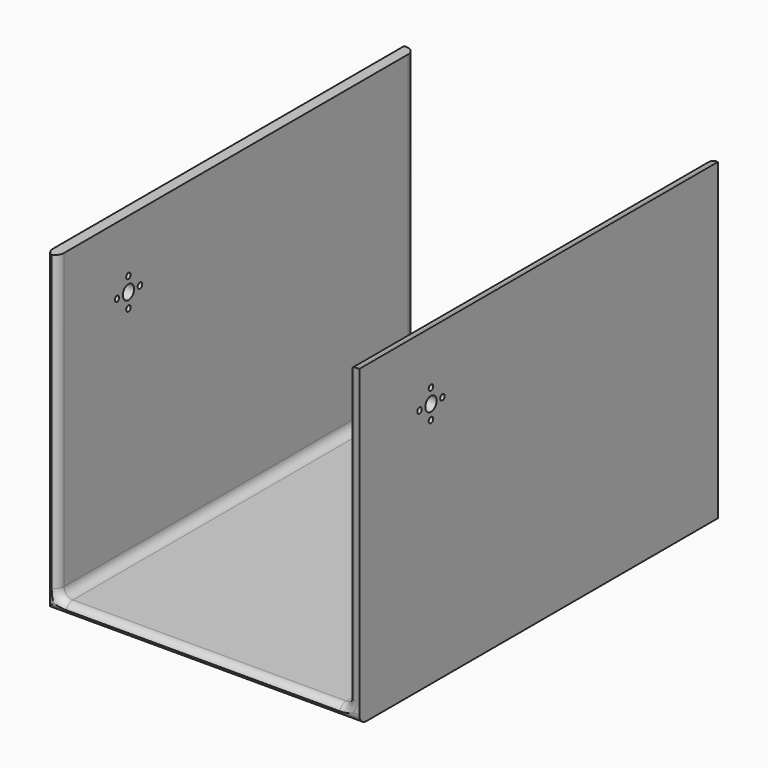
from build123d import *

# Parameters (mm, degrees)
F1_DEPTH     = 254
F2_T1_DEPTH  = 254
F2_T3_DEPTH  = 203.2
F2_T5_DEPTH  = 179.07
F2_T7_DEPTH  = 279.4
F2_T9_DEPTH  = 154.94
F2_T11_DEPTH = 203.2
F2_T14_ANGLE = 90
F2_T16_ANGLE = 90
F2_T18_ANGLE = 90
F2_T20_ANGLE = 90
F3_R         = 4.0000047
F3_R_2       = 1.5875
F4_DEPTH     = 203.2


# Not quite as in the source:
# - a fillet or chamfer that OpenCascade refuses, or shapes differently, is made with other operations: its cross-section is extruded or revolved along the edge and cut away or added


with BuildPart() as f1:
    # F0 (on Front) → F1 (new body)
    with BuildSketch(Plane.XZ):
        Polygon((-88.9, -88.9), (88.9, -88.9), (88.9, 88.9), (82.55, 88.9), (82.55, -82.55), (-82.55, -82.55), (-82.55, 88.9), (-88.9, 88.9), align=None)
    extrude(amount=F1_DEPTH)

    # F2: fillet of radius 5.08 on 11 edges, made by hand

    # F2_s2 → F2_t1 (join)
    with BuildSketch(Plane.XZ):
        with BuildLine():
            ThreePointArc((82.55, -77.47), (81.0621024484, -81.0621024484), (77.47, -82.55))
            Line((77.47, -82.55), (82.55, -82.55))
            Line((82.55, -82.55), (82.55, -77.47))
        make_face()
        with BuildLine():
            ThreePointArc((-77.47, -82.55), (-81.0621024484, -81.0621024484), (-82.55, -77.47))
            Line((-82.55, -77.47), (-82.55, -82.55))
            Line((-82.55, -82.55), (-77.47, -82.55))
        make_face()
    extrude(amount=F2_T1_DEPTH)

    # F2_s4 → F2_t3 (cut)
    with BuildSketch(Plane.YZ.offset(-101.6)):
        with BuildLine():
            ThreePointArc((-254, -83.82), (-252.5121024484, -87.4121024484), (-248.92, -88.9))
            Line((-248.92, -88.9), (-254, -88.9))
            Line((-254, -88.9), (-254, -83.82))
        make_face()
    extrude(amount=F2_T3_DEPTH, mode=Mode.SUBTRACT)

    # F2_s6 → F2_t5 (cut)
    with BuildSketch(Plane.XY.offset(-77.47)):
        with BuildLine():
            ThreePointArc((-82.55, -248.92), (-84.0378975516, -252.5121024484), (-87.63, -254))
            Line((-87.63, -254), (-82.55, -254))
            Line((-82.55, -254), (-82.55, -248.92))
        make_face()
        with BuildLine():
            ThreePointArc((87.63, 0), (84.0378975516, -1.4878975516), (82.55, -5.08))
            Line((82.55, -5.08), (82.55, 0))
            Line((82.55, 0), (87.63, 0))
        make_face()
        with BuildLine():
            ThreePointArc((87.63, -254), (84.0378975516, -252.5121024484), (82.55, -248.92))
            Line((82.55, -248.92), (82.55, -254))
            Line((82.55, -254), (87.63, -254))
        make_face()
        with BuildLine():
            ThreePointArc((-82.55, -5.08), (-84.0378975516, -1.4878975516), (-87.63, 0))
            Line((-87.63, 0), (-82.55, 0))
            Line((-82.55, 0), (-82.55, -5.08))
        make_face()
    extrude(amount=F2_T5_DEPTH, mode=Mode.SUBTRACT)

    # F2_s8 → F2_t7 (cut)
    with BuildSketch(Plane.XZ.offset(-12.7)):
        with BuildLine():
            ThreePointArc((87.63, 88.9), (84.0378975516, 87.4121024484), (82.55, 83.82))
            Line((82.55, 83.82), (82.55, 88.9))
            Line((82.55, 88.9), (87.63, 88.9))
        make_face()
    extrude(amount=F2_T7_DEPTH, mode=Mode.SUBTRACT)

    # F2_s10 → F2_t9 (cut)
    with BuildSketch(Plane.YZ.offset(-77.47)):
        with BuildLine():
            ThreePointArc((0, -87.63), (-1.4878975516, -84.0378975516), (-5.08, -82.55))
            Line((-5.08, -82.55), (0, -82.55))
            Line((0, -82.55), (0, -87.63))
        make_face()
        with BuildLine():
            ThreePointArc((-254, -87.63), (-252.5121024484, -84.0378975516), (-248.92, -82.55))
            Line((-248.92, -82.55), (-254, -82.55))
            Line((-254, -82.55), (-254, -87.63))
        make_face()
    extrude(amount=F2_T9_DEPTH, mode=Mode.SUBTRACT)

    # F2_s12 → F2_t11 (cut)
    with BuildSketch(Plane.XY.offset(-101.6)):
        with BuildLine():
            ThreePointArc((-88.9, -248.92), (-87.4121024484, -252.5121024484), (-83.82, -254))
            Line((-83.82, -254), (-88.9, -254))
            Line((-88.9, -254), (-88.9, -248.92))
        make_face()
    extrude(amount=F2_T11_DEPTH, mode=Mode.SUBTRACT)

    # F2_s13 → F2_t14 (revolve, cut)
    with BuildSketch(Plane.YZ.offset(-77.47)):
        with BuildLine():
            ThreePointArc((0, -87.63), (-1.4878975516, -84.0378975516), (-5.08, -82.55))
            Line((-5.08, -82.55), (0, -82.55))
            Line((0, -82.55), (0, -87.63))
        make_face()
    revolve(axis=Axis((-77.47, 0, -77.47), (0, 1, 0)), revolution_arc=F2_T14_ANGLE, mode=Mode.SUBTRACT)

    # F2_s15 → F2_t16 (revolve, cut)
    with BuildSketch(Plane.XY.offset(-77.47)):
        with BuildLine():
            ThreePointArc((87.63, -254), (84.0378975516, -252.5121024484), (82.55, -248.92))
            Line((82.55, -248.92), (82.55, -254))
            Line((82.55, -254), (87.63, -254))
        make_face()
    revolve(axis=Axis((77.47, -254, -77.47), (0, 1, 0)), revolution_arc=F2_T16_ANGLE, mode=Mode.SUBTRACT)

    # F2_s17 → F2_t18 (revolve, cut)
    with BuildSketch(Plane.YZ.offset(-77.47)):
        with BuildLine():
            ThreePointArc((-254, -87.63), (-252.5121024484, -84.0378975516), (-248.92, -82.55))
            Line((-248.92, -82.55), (-254, -82.55))
            Line((-254, -82.55), (-254, -87.63))
        make_face()
    revolve(axis=Axis((-77.47, -254, -77.47), (0, 1, 0)), revolution_arc=F2_T18_ANGLE, mode=Mode.SUBTRACT)

    # F2_s19 → F2_t20 (revolve, cut)
    with BuildSketch(Plane.XY.offset(-77.47)):
        with BuildLine():
            ThreePointArc((87.63, 0), (84.0378975516, -1.4878975516), (82.55, -5.08))
            Line((82.55, -5.08), (82.55, 0))
            Line((82.55, 0), (87.63, 0))
        make_face()
    revolve(axis=Axis((77.47, 0, -77.47), (0, 1, 0)), revolution_arc=F2_T20_ANGLE, mode=Mode.SUBTRACT)

    # F3 (on face) → F4 (cut)
    with BuildSketch(Plane(origin=(-88.9, 0, 0), x_dir=(0, -1, 0), z_dir=(-1, 0, 0))):
        with Locations((203.2, 50.8)):
            Circle(F3_R)
        with Locations((211.328, 50.8)):
            Circle(F3_R_2)
        with Locations((203.2, 42.672)):
            Circle(F3_R_2)
        with Locations((195.072, 50.8)):
            Circle(F3_R_2)
        with Locations((203.2, 58.928)):
            Circle(F3_R_2)
    extrude(amount=-F4_DEPTH, mode=Mode.SUBTRACT)


solid = f1.part
